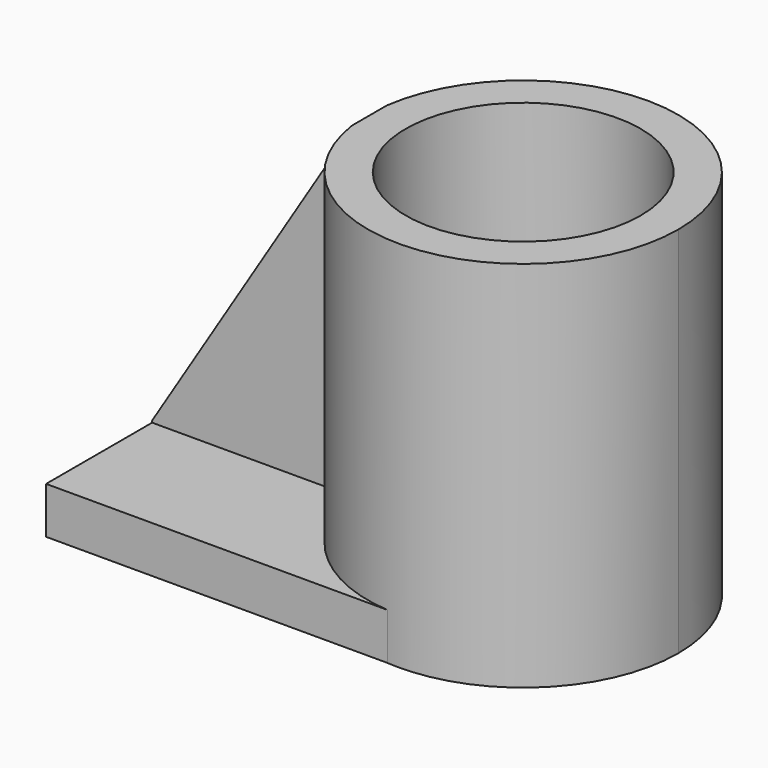
from build123d import *
from build123d import SkipClean  # not in build123d's __all__

# Parameters (mm, degrees)
F0_R     = 42.2654661293
F1_DEPTH = 101.6
F2_W     = 99.4848832185
F2_H     = 84.4806035552
F3_DEPTH = 12.7
F4_R     = 31.9997887228
F5_DEPTH = 101.601
F6_W     = 54.3876717536
F6_H     = 11.9783656307
F7_DEPTH = 101.6
F9_DEPTH = 48.3780729043


with BuildPart() as f1:
    # F0 (on Top) → F1 (new body)
    with BuildSketch(Plane.XY):
        with Locations((62.4748729169, 0)):
            Circle(F0_R)
    extrude(amount=F1_DEPTH)

    # F2 (on face) → F3 (join)
    with BuildSketch(Plane(origin=(0, 0, 0), x_dir=(1, 0, 0), z_dir=(0, 0, -1))):
        with Locations((15.9839019028, -0.1000886066)):
            Rectangle(F2_W, F2_H)
    extrude(amount=-F3_DEPTH)

    # F4 (on face) → F5 (cut, through all)
    with BuildSketch(Plane.XY.offset(101.6)):
        with Locations((62.4748729169, 0)):
            Circle(F4_R)
    extrude(amount=-F5_DEPTH, mode=Mode.SUBTRACT)

    # F6 (on face) → F7 (join)
    with BuildSketch(Plane.XY.offset(12.7)):
        with Locations((-6.5647038297, -0.0474997047)):
            Rectangle(F6_W, F6_H)
    with SkipClean():  # cleaning this boolean's faces spoils the solid; the shape is the same uncleaned
        extrude(amount=F7_DEPTH)

    # F8 (on face) → F9 (cut, through all)
    with BuildSketch(Plane.XZ.offset(6.0366825201)):
        Polygon((-33.7585397065, 13.207843317), (20.6291320471, 100.9798197685), (20.6291320471, 114.3), (-33.7585397065, 114.3), align=None)
    with SkipClean():  # cleaning this boolean's faces spoils the solid; the shape is the same uncleaned
        extrude(amount=-F9_DEPTH, mode=Mode.SUBTRACT)


solid = f1.part
